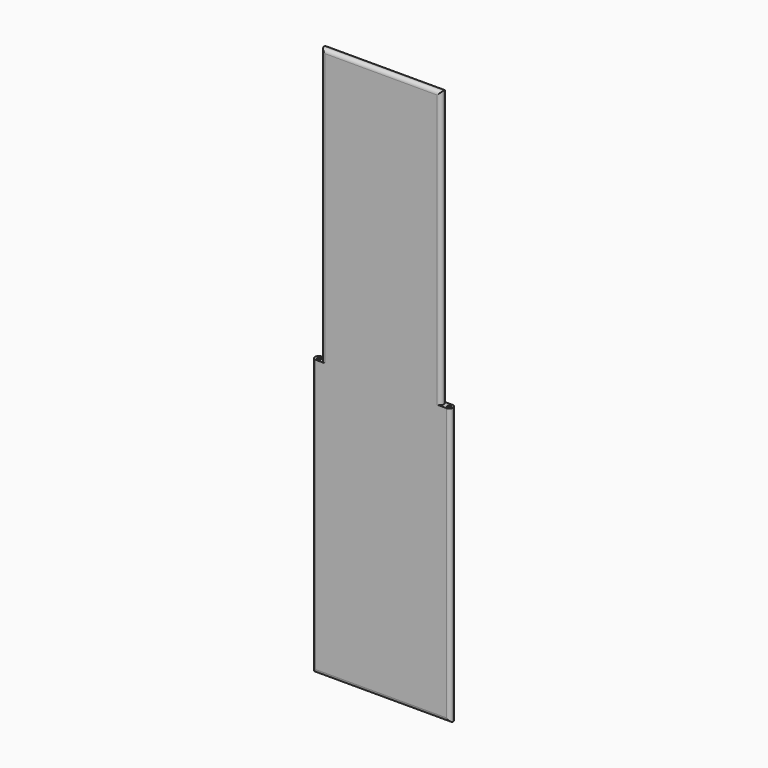
from build123d import *

# Parameters (mm, degrees)
F1_DEPTH    = 4
F2_R        = 1
F3_DEPTH    = 160.54546
F4_T1_DEPTH = 160
F4_T3_DEPTH = 155
F4_T5_DEPTH = 75
F4_T7_DEPTH = 85
F5_R        = 1
F6_DEPTH    = 158.34369
F8_DEPTH    = 1


# Not quite as in the source:
# - a fillet or chamfer that OpenCascade refuses, or shapes differently, is made with other operations: its cross-section is extruded or revolved along the edge and cut away or added


with BuildPart() as f1:
    # F0 (on Front) → F1 (new body)
    with BuildSketch(Plane.XZ):
        Polygon((-75, -3.9577843381), (-75, -153.9577843381), (0, -153.9577843381), (0, -3.9577843381), (-5, -3.9577843381), (-5, 146.0422156619), (-70, 146.0422156619), (-70, -3.9577843381), align=None)
    extrude(amount=F1_DEPTH)

    # F2 (on face) → F3 (cut)
    with BuildSketch(Plane.XY.offset(-3.9577843381)):
        with Locations((-72.5, -2)):
            Circle(F2_R)
    extrude(amount=-F3_DEPTH, mode=Mode.SUBTRACT)

    # F4: fillet of radius 2 on 12 edges, made by hand

    # F4_s2 → F4_t1 (cut)
    with BuildSketch(Plane.XY.offset(-158.9577843381)):
        with BuildLine():
            ThreePointArc((-73, -4), (-74.4142135624, -3.4142135624), (-75, -2))
            Line((-75, -2), (-75, -4))
            Line((-75, -4), (-73, -4))
        make_face()
        with BuildLine():
            ThreePointArc((-73, 0), (-74.4142135624, -0.5857864376), (-75, -2))
            Line((-75, -2), (-75, 0))
            Line((-75, 0), (-73, 0))
        make_face()
        with BuildLine():
            ThreePointArc((-2, 0), (-0.5857864376, -0.5857864376), (0, -2))
            Line((0, -2), (0, 0))
            Line((0, 0), (-2, 0))
        make_face()
        with BuildLine():
            ThreePointArc((-2, -4), (-0.5857864376, -3.4142135624), (0, -2))
            Line((0, -2), (0, -4))
            Line((0, -4), (-2, -4))
        make_face()
    extrude(amount=F4_T1_DEPTH, mode=Mode.SUBTRACT)

    # F4_s4 → F4_t3 (cut)
    with BuildSketch(Plane.XY.offset(-3.9577843381)):
        with BuildLine():
            ThreePointArc((-68, -4), (-69.4142135624, -3.4142135624), (-70, -2))
            Line((-70, -2), (-70, -4))
            Line((-70, -4), (-68, -4))
        make_face()
        with BuildLine():
            ThreePointArc((-68, 0), (-69.4142135624, -0.5857864376), (-70, -2))
            Line((-70, -2), (-70, 0))
            Line((-70, 0), (-68, 0))
        make_face()
        with BuildLine():
            ThreePointArc((-5, -2), (-5.5857864376, -0.5857864376), (-7, 0))
            Line((-7, 0), (-5, 0))
            Line((-5, 0), (-5, -2))
        make_face()
        with BuildLine():
            ThreePointArc((-5, -2), (-5.5857864376, -3.4142135624), (-7, -4))
            Line((-7, -4), (-5, -4))
            Line((-5, -4), (-5, -2))
        make_face()
    extrude(amount=F4_T3_DEPTH, mode=Mode.SUBTRACT)

    # F4_s6 → F4_t5 (cut)
    with BuildSketch(Plane.YZ.offset(-75)):
        with BuildLine():
            ThreePointArc((-2, 146.0422156619), (-3.4142135624, 145.4564292243), (-4, 144.0422156619))
            Line((-4, 144.0422156619), (-4, 146.0422156619))
            Line((-4, 146.0422156619), (-2, 146.0422156619))
        make_face()
        with BuildLine():
            ThreePointArc((-2, 146.0422156619), (-0.5857864376, 145.4564292243), (0, 144.0422156619))
            Line((0, 144.0422156619), (0, 146.0422156619))
            Line((0, 146.0422156619), (-2, 146.0422156619))
        make_face()
    extrude(amount=F4_T5_DEPTH, mode=Mode.SUBTRACT)

    # F4_s8 → F4_t7 (cut)
    with BuildSketch(Plane.YZ.offset(-80)):
        with BuildLine():
            ThreePointArc((-4, -151.9577843381), (-3.4142135624, -153.3719979004), (-2, -153.9577843381))
            Line((-2, -153.9577843381), (-4, -153.9577843381))
            Line((-4, -153.9577843381), (-4, -151.9577843381))
        make_face()
        with BuildLine():
            ThreePointArc((0, -151.9577843381), (-0.5857864376, -153.3719979004), (-2, -153.9577843381))
            Line((-2, -153.9577843381), (0, -153.9577843381))
            Line((0, -153.9577843381), (0, -151.9577843381))
        make_face()
    extrude(amount=F4_T7_DEPTH, mode=Mode.SUBTRACT)

    # F5 (on face) → F6 (cut)
    with BuildSketch(Plane.XY.offset(-3.9577843381)):
        with Locations((-2, -2)):
            Circle(F5_R)
    extrude(amount=-F6_DEPTH, mode=Mode.SUBTRACT)

    # F7 (on face) → F8 (join)
    with BuildSketch(Plane(origin=(0, 0, 0), x_dir=(-1, 0, 0), z_dir=(0, 1, 0))):
        with BuildLine():
            Line((57.5, 127.8843627218), (17.5, 127.8843627218))
            Line((17.5, 127.8843627218), (17.5, 119.8843627218))
            ThreePointArc((17.5, 119.8843627218), (37.5, 99.8843627218), (57.5, 119.8843627218))
            Line((57.5, 119.8843627218), (57.5, 127.8843627218))
        make_face()
        with BuildLine():
            Line((25.5, 119.8843627218), (49.5, 119.8843627218))
            ThreePointArc((49.5, 119.8843627218), (37.5, 107.8843627218), (25.5, 119.8843627218))
        make_face(mode=Mode.SUBTRACT)
        with BuildLine():
            Line((57.5, 95.1502709985), (17.5, 95.1502709985))
            Line((17.5, 95.1502709985), (17.5, 87.1502709985))
            Line((17.5, 87.1502709985), (37.5, 87.1502709985))
            Line((37.5, 87.1502709985), (17.5, 78.7390248019))
            Line((17.5, 78.7390248019), (17.5, 70.7390248019))
            Line((17.5, 70.7390248019), (37.5, 79.1502709985))
            ThreePointArc((37.5, 79.1502709985), (48.4049875621, 71.1003953774), (57.5, 81.1502709985))
            Line((57.5, 81.1502709985), (57.5, 87.1502709985))
            Line((57.5, 87.1502709985), (57.5, 95.1502709985))
        make_face()
        with BuildLine():
            Line((43.5, 87.1502709985), (51.5, 87.1502709985))
            Line((51.5, 87.1502709985), (51.5, 81.1502709985))
            ThreePointArc((51.5, 81.1502709985), (47.5, 77.1502709985), (43.5, 81.1502709985))
            Line((43.5, 81.1502709985), (43.5, 87.1502709985))
        make_face(mode=Mode.SUBTRACT)
        Polygon((57.5, 53.6148357394), (17.5, 66.7390248019), (17.5, 58.7390248019), (31.5839202169, 53.6984175146), (31.5839202169, 45.6984175146), (17.5, 40.7758287685), (17.5, 32.7758287685), (57.5, 45.6148357394), align=None)
        Polygon((37.5, 52.6984175146), (49.1189500386, 49.6984175146), (37.5, 46.6984175146), align=None, mode=Mode.SUBTRACT)
        Polygon((57.5, 28.7758287685), (17.5, 28.7758287685), (17.5, 20.7758287685), (33.5, 20.7758287685), (33.5, 11.7758287685), (41.5, 11.7758287685), (41.5, 20.7758287685), (49.5, 20.7758287685), (49.5, 4.7758287685), (57.5, 4.7758287685), align=None)
        Polygon((57.5, -23.2241712315), (57.5, 0.7758287685), (49.5, 0.7758287685), (49.5, -7.2241712315), (17.5, -7.2241712315), (17.5, -15.2241712315), (49.5, -15.2241712315), (49.5, -23.2241712315), align=None)
        Polygon((57.5, -35.2241712315), (57.5, -27.2241712315), (17.5, -27.2241712315), (17.4124501646, -35.2241712315), align=None)
        Polygon((57.5, -47.2241712315), (57.5, -39.2241712315), (17.5, -39.2241712315), (17.5, -47.2241712315), (41.5822874359, -47.2241712315), (17.5, -61.2241712315), (17.5, -69.2241712315), (57.5, -69.2241712315), (57.5, -61.2241712315), (33.4177125641, -61.2241712315), align=None)
        with BuildLine():
            Line((41.5, -97.2241712315), (41.5, -103.2241712315))
            ThreePointArc((41.5, -103.2241712315), (56.5, -88.2241712315), (41.5, -73.2241712315))
            Line((41.5, -73.2241712315), (33.5, -73.2241712315))
            ThreePointArc((33.5, -73.2241712315), (18.5, -88.2241712315), (33.5, -103.2241712315))
            Line((33.5, -103.2241712315), (33.5, -97.2241712315))
            ThreePointArc((33.5, -97.2241712315), (30.288601192, -96.6317224622), (27.5, -94.932375164))
            ThreePointArc((27.5, -94.932375164), (25.0924487693, -85.0127724236), (33.5, -79.2241712315))
            Line((33.5, -79.2241712315), (41.5, -79.2241712315))
            ThreePointArc((41.5, -79.2241712315), (50.5, -88.2241712315), (41.5, -97.2241712315))
        make_face()
        with BuildLine():
            ThreePointArc((27.5, -94.932375164), (30.288601192, -96.6317224622), (33.5, -97.2241712315))
            Line((33.5, -97.2241712315), (33.5, -88.2241712315))
            Line((33.5, -88.2241712315), (27.5, -88.2241712315))
            Line((27.5, -88.2241712315), (27.5, -94.932375164))
        make_face()
    extrude(amount=F8_DEPTH)


solid = f1.part
